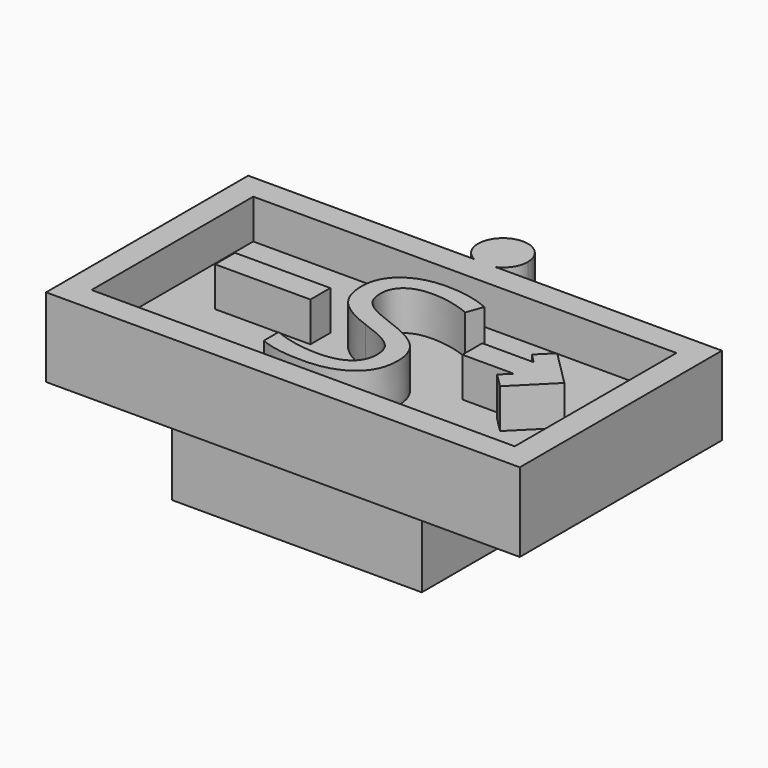
from build123d import *

# Parameters (mm, degrees)
F1_DEPTH     = 3.175
F2_W         = 17.018
F2_H         = 8.128
F3_DEPTH     = 1.5875
F4_W         = 10.05
F4_H         = 8.76
F5_DEPTH     = 3
F6_R         = 3.5
F7_DEPTH     = 3.5
F8_W         = 3.8331345095
F8_H         = 1
F8_TEXT_SIZE = 9.2277777778
F9_DEPTH     = 1.5875


# Not quite as in the source:
# - ends of sketch curves that miss each other by under 0.0002 mm in the source are joined
# - Text() gives the source's letters only with a copy of the font that has no kerning and outlines rounded to 1/6400 em; it was checked with that copy


with BuildPart() as f1:
    # F0 (on Top) → F1 (new body)
    with BuildSketch(Plane.XY):
        with BuildLine():
            Line((-9.9608898944, 10.16), (-19.05, 10.16))
            Line((-19.05, 10.16), (-19.05, 0))
            Line((-19.05, 0), (0, 0))
            Line((0, 0), (0, 10.16))
            Line((0, 10.16), (-9.0891101056, 10.16))
            ThreePointArc((-9.0891101056, 10.16), (-9.525, 10.06), (-9.9608898944, 10.16))
        make_face()
        with BuildLine():
            ThreePointArc((-8.525, 11.06), (-10.0560885546, 11.9073163206), (-9.9608898944, 10.16))
            Line((-9.9608898944, 10.16), (-9.0891101056, 10.16))
            ThreePointArc((-9.0891101056, 10.16), (-8.6776836794, 10.5289114454), (-8.525, 11.06))
        make_face()
        with BuildLine():
            Line((-9.0891101056, 10.16), (-9.9608898944, 10.16))
            ThreePointArc((-9.9608898944, 10.16), (-9.525, 10.06), (-9.0891101056, 10.16))
        make_face()
    extrude(amount=F1_DEPTH)

    # F2 (on face) → F3 (cut)
    with BuildSketch(Plane.XY.offset(3.175)):
        with Locations((-9.525, 5.08)):
            Rectangle(F2_W, F2_H)
    extrude(amount=-F3_DEPTH, mode=Mode.SUBTRACT)

    # F4 (on face) → F5 (join)
    with BuildSketch(Plane(origin=(0, 0, 0), x_dir=(1, 0, 0), z_dir=(0, 0, -1))):
        with Locations((-9.525, -5.08)):
            Rectangle(F4_W, F4_H)
    extrude(amount=F5_DEPTH)

    # F6 (on face) → F7 (cut)
    with BuildSketch(Plane(origin=(0, 0, -3), x_dir=(1, 0, 0), z_dir=(0, 0, -1))):
        with Locations((-9.525, -5.08)):
            Circle(F6_R)
    extrude(amount=-F7_DEPTH, mode=Mode.SUBTRACT)

    # F8 (on face) → F9 (join, through all)
    with BuildSketch(Plane.XY.offset(1.5875)):
        with Locations((-14.1792780978, 5.3028898657)):
            Rectangle(F8_W, F8_H)
        Polygon((-4.1229840255, 5.8529416598), (-6.1898453526, 5.8529416598), (-6.1898453526, 4.8529416598), (-4.1229840255, 4.8529416598), (-4.4943519679, 4.4815726779), (-3.928666543, 3.915887253), (-2.4916126558, 5.3529411401), (-3.928666543, 6.7899950272), (-4.4943519679, 6.2243096023), align=None)
        with Locations((-12.1354518229, 1.5)):
            Text('S', F8_TEXT_SIZE, font='Open Sans', text_align=(TextAlign.LEFT, TextAlign.BOTTOM))
    extrude(amount=F9_DEPTH)


solid = f1.part
